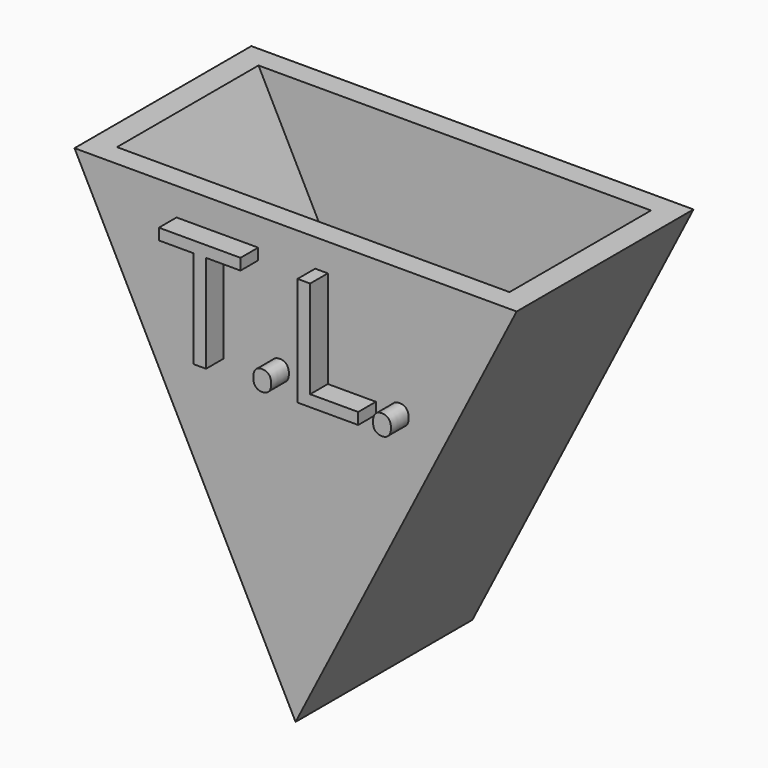
from build123d import *

# Parameters (mm, degrees)
F1_DEPTH     = 25.4
F2_T         = -2.54
F3_TEXT_SIZE = 17.5264263008
F4_DEPTH     = 2.54


# Not quite as in the source:
# - Text() gives the source's letters only with a copy of the font that has no kerning and outlines rounded to 1/6400 em; it was checked with that copy


with BuildPart() as f1:
    # F0 (on Front) → F1 (new body)
    with BuildSketch(Plane.XZ):
        Polygon((0, 0), (0, -49.7736315734), (25.4, 0), align=None)
        Polygon((0, 0), (-25.4, 0), (0, -49.7736315734), align=None)
    extrude(amount=F1_DEPTH)

    # F2
    f2_openings = [f1.faces().sort_by_distance(p)[0] for p in [
        (0, -12.7, 0),
    ]]
    offset(amount=F2_T, openings=f2_openings)

    # F3 (on face) → F4 (join)
    with BuildSketch(Plane.XZ.offset(25.4)):
        with Locations((-13.8272317126, -15.7066611573)):
            Text('T.L.', F3_TEXT_SIZE, font='Open Sans', text_align=(TextAlign.LEFT, TextAlign.BOTTOM))
    extrude(amount=F4_DEPTH)


solid = f1.part
